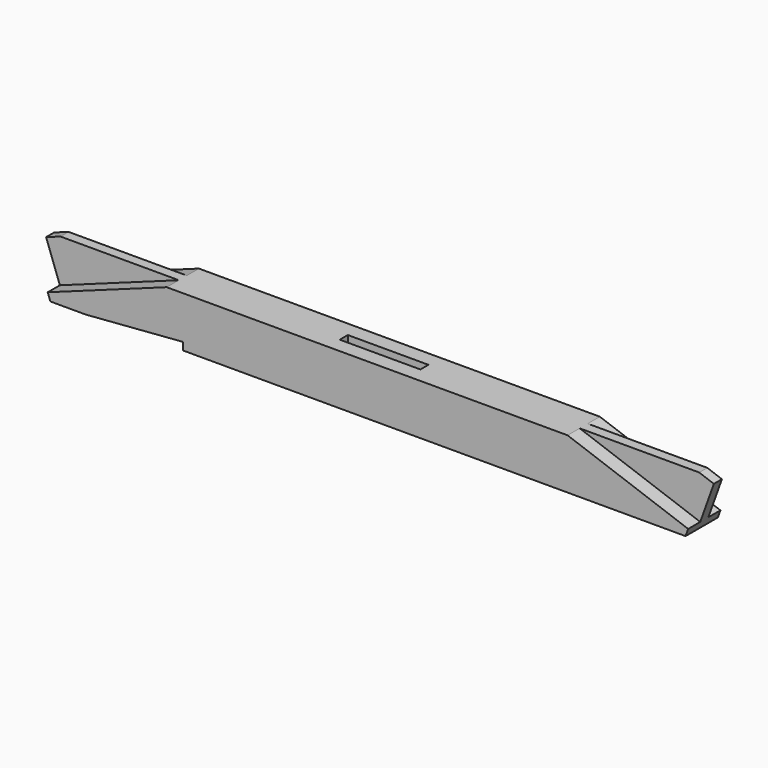
from build123d import *

# Parameters (mm, degrees)
F1_DEPTH = 101.6
F2_DEPTH = 25.4
F3_W     = 406.4
F3_H     = 50.8
F4_DEPTH = 203.2
F5_W     = 488.4674
F5_H     = 38.1
F6_DEPTH = 88.9
F8_DEPTH = 203.2


# Not quite as in the source:
# - a feature names something its author has since deleted; it is built from what else it names


with BuildPart() as f1:
    # F0 (on Front) → F1 (new body, symmetric)
    with BuildSketch(Plane.XZ):
        Polygon((-1613.4907807573, -90.3599756084), (-1600.2, -127), (1600.2, -127), (1613.2038848964, -90.7061572542), (1072.3230234564, 103.0884903417), (1005.586, 127), (-1014.2728, 127), (-1080.098633757, 103.1223760313), align=None)
    extrude(amount=F1_DEPTH, both=True)

    # F0 (on Front) → F2 (join, symmetric)
    with BuildSketch(Plane.XZ):
        Polygon((-1088.7599889401, 127), (-1610.1703115208, 127), (-1682.781622222, 100.6610161415), (-1613.4907807573, -90.3599756084), (-1080.098633757, 103.1223760313), align=None)
        Polygon((1072.3230234564, 103.0884903417), (1613.2038848964, -90.7061572542), (1681.7427875358, 100.5859200125), (1608.0210902906, 127), (1080.8903862863, 127), align=None)
        Polygon((1080.8903862863, 127), (1005.586, 127), (1072.3230234564, 103.0884903417), align=None)
        Polygon((-1014.2728, 127), (-1088.7599889401, 127), (-1080.098633757, 103.1223760313), align=None)
    extrude(amount=F2_DEPTH, both=True)

    # F3 (on face) → F4 (cut)
    with BuildSketch(Plane.XY.offset(127)):
        Rectangle(F3_W, F3_H)
    extrude(amount=-F4_DEPTH, mode=Mode.SUBTRACT)

    # F5 (on face) → F6 (cut)
    with BuildSketch(Plane(origin=(0, 0, -127), x_dir=(1, 0, 0), z_dir=(0, 0, -1))):
        with Locations((-1175.5755, 0)):
            Rectangle(F5_W, F5_H)
    extrude(amount=-F6_DEPTH, mode=Mode.SUBTRACT)

    # F7 (on face) → F8 (cut)
    with BuildSketch(Plane.XZ.offset(101.6)):
        Polygon((-1421.4916229248, -127), (-931.272983551, -127), (-931.272983551, -88.9), align=None)
    extrude(amount=-F8_DEPTH, mode=Mode.SUBTRACT)


solid = f1.part
